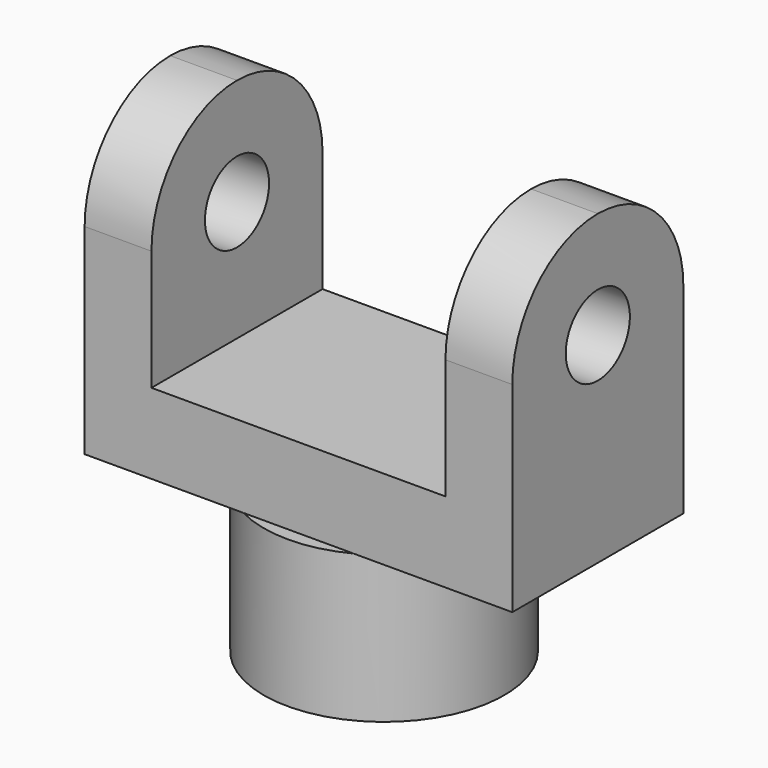
from build123d import *

# Parameters (mm, degrees)
F0_W     = 9
F0_H     = 11
F2_DEPTH = 8
F4_DEPTH = 11
F5_R     = 3
F6_DEPTH = 32.001


# Not quite as in the source:
# - a feature names something its author has since deleted; it is built from what else it names


with BuildPart() as f1:
    # F0 (on Front) → F1 (revolve)
    with BuildSketch(Plane.XZ):
        with Locations((11.5, -5.5)):
            Rectangle(F0_W, F0_H)
    revolve(axis=Axis((16, 0, -5.5), (0, 0, -1)))

    # F0 (on Front) → F2 (join, symmetric)
    with BuildSketch(Plane.XZ):
        Polygon((0, 23), (0, 0), (7, 0), (16, 0), (32, 0), (32, 23), (27, 23), (27, 6), (5, 6), (5, 23), align=None)
    extrude(amount=F2_DEPTH, both=True)

    # F3 (on face) → F4 (cut)
    with BuildSketch(Plane(origin=(0, 0, -11), x_dir=(1, 0, 0), z_dir=(0, 0, -1))):
        with BuildLine():
            Line((14.5, 6.2696960071), (14.5, 4.7696960071))
            ThreePointArc((14.5, 4.7696960071), (16, -5), (17.5, 4.7696960071))
            Line((17.5, 4.7696960071), (17.5, 6.2696960071))
            Line((17.5, 6.2696960071), (14.5, 6.2696960071))
        make_face()
    extrude(amount=-F4_DEPTH, mode=Mode.SUBTRACT)

    # F5 (on face) → F6 (cut, through all)
    with BuildSketch(Plane.YZ.offset(32)):
        with Locations((0, 15)):
            Circle(F5_R)
        with BuildLine():
            ThreePointArc((-8, 15), (-5.6568542495, 20.6568542495), (0, 23))
            Line((0, 23), (-8, 23))
            Line((-8, 23), (-8, 15))
        make_face()
        with BuildLine():
            ThreePointArc((0, 23), (5.6568542495, 20.6568542495), (8, 15))
            Line((8, 15), (8, 23))
            Line((8, 23), (0, 23))
        make_face()
    extrude(amount=-F6_DEPTH, mode=Mode.SUBTRACT)


solid = f1.part
